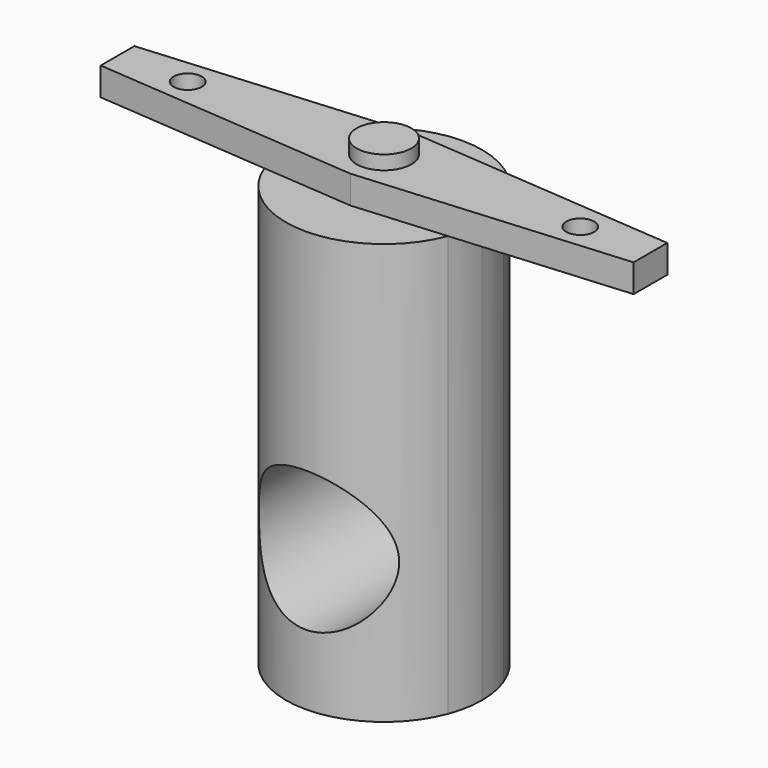
from build123d import *

# Parameters (mm, degrees)
F0_R     = 1
F1_DEPTH = 2
F2_R     = 1.95
F3_DEPTH = 1
F5_DEPTH = 30
F6_R     = 5
F7_DEPTH = 12.5


# Not quite as in the source:
# - ends of sketch curves that miss each other by under 0.0002 mm in the source are joined


with BuildPart() as f1:
    # F0 (on Top) → F1 (new body)
    with BuildSketch(Plane.XY):
        Polygon((0, -3), (0, 0), (0, 3), (-19, 1.5), (-19, 0), (-19, -1.5), align=None)
        with Locations((-14, 0)):
            Circle(F0_R, mode=Mode.SUBTRACT)
        Polygon((0, 3), (0, 0), (0, -3), (18.9999993891, -1.5), (18.9999993891, 0), (18.9999993891, 1.5), align=None)
        with Locations((14, 0)):
            Circle(F0_R, mode=Mode.SUBTRACT)
    extrude(amount=F1_DEPTH)

    # F2 (on face) → F3 (join)
    with BuildSketch(Plane.XY.offset(2)):
        Circle(F2_R)
    extrude(amount=F3_DEPTH)

    # F4 (on face) → F5 (join)
    with BuildSketch(Plane(origin=(0, 0, 0), x_dir=(1, 0, 0), z_dir=(0, 0, -1))):
        with BuildLine():
            Line((0, 3), (6.5447045484, 2.4833127822))
            ThreePointArc((6.5447045484, 2.4833127822), (9.2e-09, 7), (-6.5447045419, 2.4833127993))
            Line((-6.5447045419, 2.4833127993), (0, 3))
        make_face()
        with BuildLine():
            ThreePointArc((6.5447045484, -2.4833127822), (6.8852353569, -1.2623525976), (7, 0))
            ThreePointArc((7, 0), (6.8852353569, 1.2623525976), (6.5447045484, 2.4833127822))
            Line((6.5447045484, 2.4833127822), (0, 3))
            Line((0, 3), (-6.5447045419, 2.4833127993))
            ThreePointArc((-6.5447045419, 2.4833127993), (-7, 0), (-6.5447045419, -2.4833127993))
            Line((-6.5447045419, -2.4833127993), (0, -3))
            Line((0, -3), (6.5447045484, -2.4833127822))
        make_face()
        with BuildLine():
            ThreePointArc((-6.5447045419, -2.4833127993), (9.2e-09, -7), (6.5447045484, -2.4833127822))
            Line((6.5447045484, -2.4833127822), (0, -3))
            Line((0, -3), (-6.5447045419, -2.4833127993))
        make_face()
    extrude(amount=F5_DEPTH)

    # F6 (on Front) → F7 (cut, symmetric)
    with BuildSketch(Plane.XZ):
        with Locations((0, -20)):
            Circle(F6_R)
    extrude(amount=F7_DEPTH, both=True, mode=Mode.SUBTRACT)


solid = f1.part
